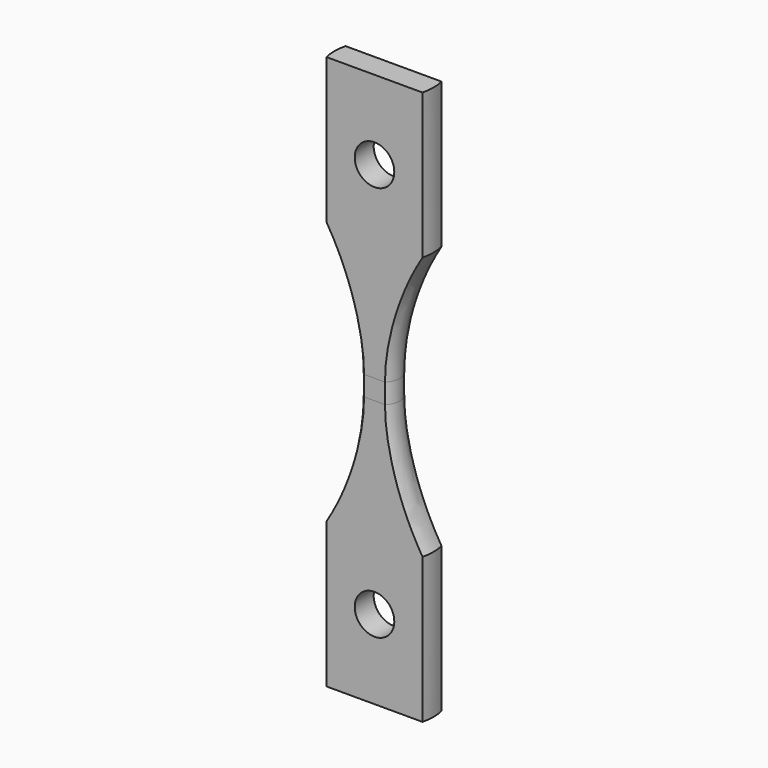
from build123d import *

# Parameters (mm, degrees)
F4_DEPTH = 0.3
F5_R     = 0.5
F6_DEPTH = 12.5


# Not quite as in the source:
# - a feature names something its author has since deleted; it is built from what else it names


with BuildPart() as f1:
    # F0 (on Front) → F1 (revolve)
    with BuildSketch(Plane.XZ):
        with BuildLine():
            Line((1.25, 7), (0, 7))
            Line((0, 7), (0, 0.25))
            Line((0, 0.25), (0.4, 0.25))
            ThreePointArc((0.4, 0.25), (0.6164025036, 1.8468719423), (1.25, 3.3285548558))
            Line((1.25, 3.3285548558), (1.25, 7))
        make_face()
    revolve(axis=Axis((0, 0, 3.5), (0, 0, -1)))


with BuildPart() as f2:
    # F0 (on Front) → F2 (revolve)
    with BuildSketch(Plane.XZ):
        Polygon((0.4, 0.25), (0, 0.25), (0, 0), (0, -0.25), (0.4, -0.25), align=None)
    revolve(axis=Axis((0, 0, 3.5), (0, 0, -1)))


with BuildPart() as f4_tool:
    # F3 (on Front) → F4 (new body, symmetric)
    with BuildSketch(Plane.XZ):
        Polygon((1.25, 0.25), (1.25, 7.75), (0, 7.75), (-1.25, 7.75), (-1.25, 0.25), (-1.25, -0.25), (0, -0.25), (1.25, -0.25), align=None)
    extrude(amount=F4_DEPTH, both=True)


with BuildPart() as f1_1:
    add(f1.part)

    # F4: intersect by f4_tool
    add(f4_tool.part, mode=Mode.INTERSECT)

    # F5 (on Front) → F6 (cut, symmetric)
    with BuildSketch(Plane.XZ):
        with Locations((0, 5)):
            Circle(F5_R)
    extrude(amount=F6_DEPTH, both=True, mode=Mode.SUBTRACT)


with BuildPart() as f2_1:
    add(f2.part)

    # F4: intersect by f4_tool
    add(f4_tool.part, mode=Mode.INTERSECT)


with BuildPart() as f7_1:
    # F7: instance of F1
    add(f1_1.part.mirror(Plane.XY))


solid = Compound([f1_1.part, f2_1.part, f7_1.part])
